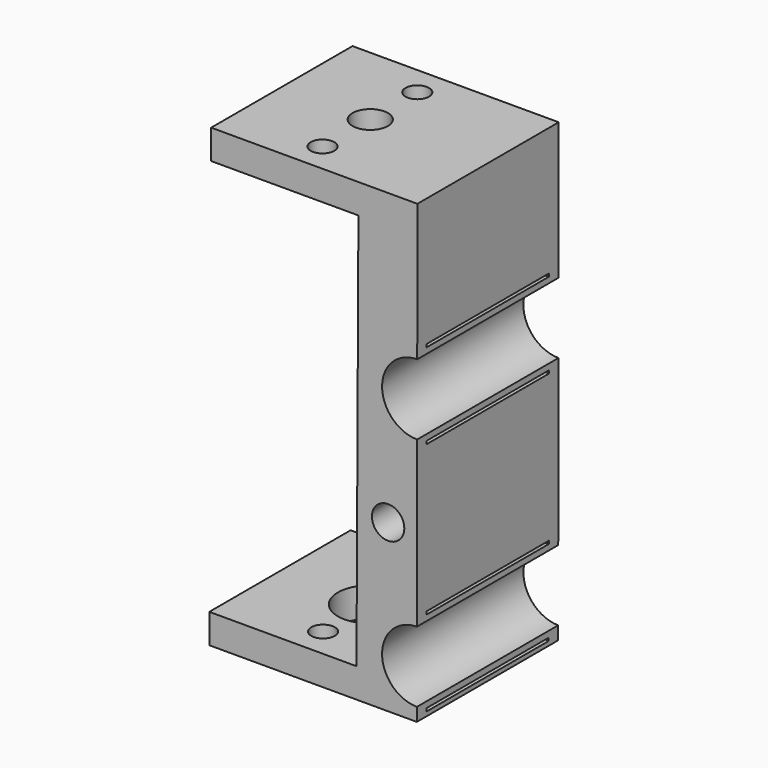
from build123d import *

# Parameters (mm, degrees)
F0_R          = 5.5
F1_DEPTH      = 60
F4_DEPTH      = 26
F4_DEPTH_BACK = 26
F5_R          = 4
F6_DEPTH      = 5
F7_R          = 4
F8_DEPTH      = 15
F9_R          = 11
F10_DEPTH     = 10.001
F11_R         = 6
F12_DEPTH     = 25


# Not quite as in the source:
# - a feature names something its author has since deleted; it is built from what else it names


with BuildPart() as f1:
    # F0 (on Front) → F1 (new body)
    with BuildSketch(Plane.XZ):
        with BuildLine():
            ThreePointArc((-0.0872969156, -53.4805140133), (-11.9999962709, -41.4659778258), (-0.0575900904, -29.4809696761))
            Line((-0.0575900904, -29.4809696761), (-5.4639e-06, 17.0404876904))
            Line((-5.4639e-06, 17.0404876904), (-70.0428405992, 17.0404876904))
            Line((-70.0428405992, 17.0404876904), (-70.0428405992, 7.0404876904))
            Line((-70.0428405992, 7.0404876904), (-20.0428405992, 7.0404876904))
            Line((-20.0428405992, 7.0404876904), (-20.6929361639, -127.9595123096))
            Line((-20.6929361639, -127.9595123096), (-70.6929361639, -127.9595123096))
            Line((-70.6929361639, -127.9595123096), (-70.6929361639, -137.9595123096))
            Line((-70.6929361639, -137.9595123096), (-0.1918656855, -137.9595123096))
            Line((-0.1918656855, -137.9595123096), (-0.1862936956, -133.4580141387))
            ThreePointArc((-0.1862936956, -133.4580141387), (-11.9988136294, -121.4446249335), (-0.1565894029, -109.4605157571))
            Line((-0.1565894029, -109.4605157571), (-0.0872969156, -53.4805140133))
        make_face()
        with Locations((-9.947382845, -81.480831509)):
            Circle(F0_R, mode=Mode.SUBTRACT)
    extrude(amount=F1_DEPTH)


with BuildPart() as f1_1:
    # F2: moved
    add(f1.part.moved(Location((0, 30, 0))))

    # F3 (on Front) → F4 (cut, two sides)
    with BuildSketch(Plane.XZ) as f4_sk:
        with BuildLine():
            ThreePointArc((0, -55.5154254436), (-14, -41.5154254436), (0, -27.5154254436))
            Line((0, -27.5154254436), (0, -26.5154254436))
            ThreePointArc((0, -26.5154254436), (-15, -41.5154254436), (0, -56.5154254436))
            Line((0, -56.5154254436), (0, -55.5154254436))
        make_face()
        with BuildLine():
            Line((0, -107.5154236555), (0, -106.5154236555))
            ThreePointArc((0, -106.5154236555), (-15, -121.5154236555), (0, -136.5154236555))
            Line((0, -136.5154236555), (0, -135.5154236555))
            ThreePointArc((0, -135.5154236555), (-14, -121.5154236555), (0, -107.5154236555))
        make_face()
    extrude(amount=F4_DEPTH, mode=Mode.SUBTRACT)
    extrude(f4_sk.sketch, amount=-F4_DEPTH_BACK, mode=Mode.SUBTRACT)

    # F5 (on face) → F6 (cut)
    with BuildSketch(Plane.XY.offset(-127.9595123096)):
        with Locations((-40.0428405992, -20)):
            Circle(F5_R)
        with Locations((-40.0428405992, 20)):
            Circle(F5_R)
    extrude(amount=-F6_DEPTH, mode=Mode.SUBTRACT)

    # F7 (on face) → F8 (cut)
    with BuildSketch(Plane.XY.offset(17.0404876904)):
        with Locations((-40.0428405992, 20)):
            Circle(F7_R)
        with Locations((-40.2286797762, -20)):
            Circle(F7_R)
    extrude(amount=-F8_DEPTH, mode=Mode.SUBTRACT)

    # F9 (on face) → F10 (cut, through all)
    with BuildSketch(Plane.XY.offset(-127.9595123096)):
        with Locations((-40.0215312839, 0)):
            Circle(F9_R)
    extrude(amount=-F10_DEPTH, mode=Mode.SUBTRACT)

    # F11 (on face) → F12 (cut)
    with BuildSketch(Plane.XY.offset(17.0404876904)):
        with Locations((-40.0154478848, 0)):
            Circle(F11_R)
    extrude(amount=-F12_DEPTH, mode=Mode.SUBTRACT)


solid = f1_1.part
